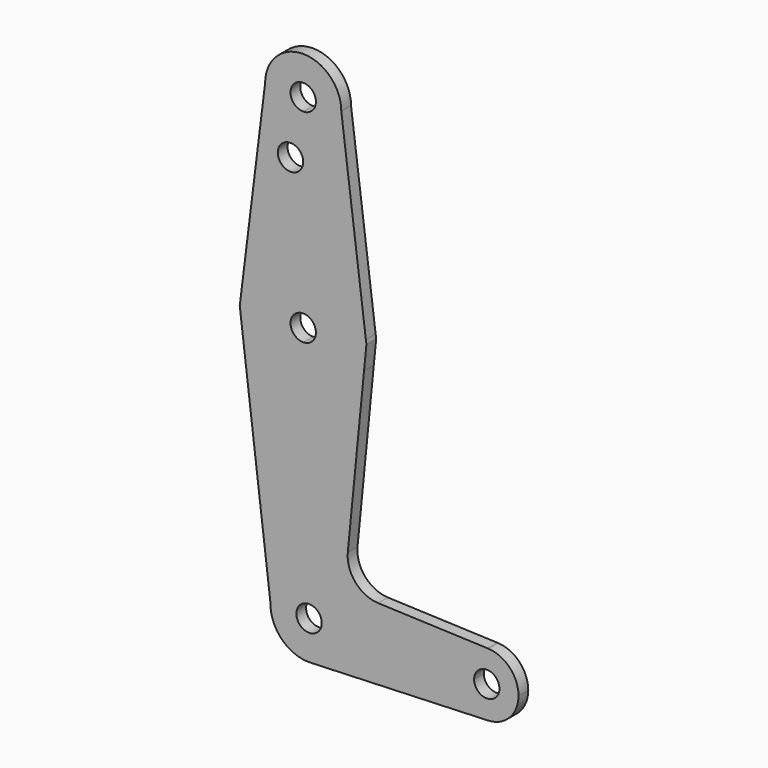
from build123d import *

# Parameters (mm, degrees)
F0_R     = 3.175
F1_DEPTH = 3.048


with BuildPart() as f1:
    # F0 (on Front) → F1 (new body)
    with BuildSketch(Plane.XZ):
        with BuildLine():
            ThreePointArc((-40.2117882118, -46.0434157276), (-37.9195183152, -46.9467537328), (-36.9635307828, -49.2175704733))
            Line((-36.9635307828, -49.2175704733), (-30.4929387527, -49.2175704733))
            ThreePointArc((-30.4929387527, -49.2175704733), (-33.3972114214, -42.3188706769), (-40.3610855146, -39.5745463105))
            Line((-40.3610855146, -39.5745463105), (-40.2117882118, -46.0434157276))
        make_face()
        with BuildLine():
            Line((-30.4929387527, -49.2175704733), (-36.9635307828, -49.2175704733))
            ThreePointArc((-36.9635307828, -49.2175704733), (-42.3575432504, -51.4883872137), (-40.2117882118, -46.0434157276))
            Line((-40.2117882118, -46.0434157276), (-40.3610855146, -39.5745463105))
            ThreePointArc((-40.3610855146, -39.5745463105), (-46.9764555291, -42.4146129712), (-49.7825692087, -49.0444564898))
            ThreePointArc((-49.7825692087, -49.0444564898), (-46.7848835913, -56.2078093787), (-39.4795413303, -58.8406250046))
            ThreePointArc((-39.4795413303, -58.8406250046), (-33.0889283464, -55.8009245652), (-30.4929387527, -49.2175704733))
        make_face()
        with BuildLine():
            ThreePointArc((-40.3610855146, -39.5745463105), (-33.3972114214, -42.3188706769), (-30.4929387527, -49.2175704733))
            Line((-30.4929387527, -49.2175704733), (-3.6260307828, -49.2175704733))
            ThreePointArc((-3.6260307828, -49.2175704733), (-1.2243575174, -43.5291147413), (4.5272992617, -41.2830053534))
            Line((4.5272992617, -41.2830053534), (-22.8459084544, -40.2300400931))
            ThreePointArc((-22.8459084544, -40.2300400931), (-28.5326050858, -37.5104766919), (-30.452220219, -31.5063429983))
            Line((-30.452220219, -31.5063429983), (-26.3874033783, 9.7581951748))
            ThreePointArc((-26.3874033783, 9.7581951748), (-31.9659630039, 1.6680517084), (-41.2377823768, -1.5883442013))
            Line((-41.2377823768, -1.5883442013), (-40.3610855146, -39.5745463105))
        make_face()
        with BuildLine():
            Line((-3.6260307828, -49.2175704733), (-30.4929387527, -49.2175704733))
            ThreePointArc((-30.4929387527, -49.2175704733), (-33.0889283464, -55.8009245652), (-39.4795413303, -58.8406250046))
            Line((-39.4795413303, -58.8406250046), (4.6157088211, -57.1492376696))
            ThreePointArc((4.6157088211, -57.1492376696), (-1.1925749502, -54.9367840602), (-3.6260307828, -49.2175704733))
        make_face()
        with BuildLine():
            ThreePointArc((-49.7825692087, -49.0444564898), (-46.9764555291, -42.4146129712), (-40.3610855146, -39.5745463105))
            Line((-40.3610855146, -39.5745463105), (-41.2377823768, -1.5883442013))
            ThreePointArc((-41.2377823768, -1.5883442013), (-51.3557623371, 1.7556537149), (-57.0797223857, 10.7440975125))
            Line((-57.0797223857, 10.7440975125), (-49.7825692087, -49.0444564898))
        make_face()
        with BuildLine():
            ThreePointArc((4.5272992617, -41.2830053534), (-1.2243575174, -43.5291147413), (-3.6260307828, -49.2175704733))
            ThreePointArc((-3.6260307828, -49.2175704733), (-1.1925749502, -54.9367840602), (4.6157088211, -57.1492376696))
            ThreePointArc((4.6157088211, -57.1492376696), (10.0306828042, -54.7216146407), (12.2489692172, -49.2175704733))
            ThreePointArc((12.2489692172, -49.2175704733), (10.0618609106, -43.7461079976), (4.705812903, -41.2898722381))
            Line((4.705812903, -41.2898722381), (4.5272992617, -41.2830053534))
        make_face()
        with BuildLine():
            ThreePointArc((7.480460495, -49.2175704733), (4.3114692172, -52.386561751), (1.1424779394, -49.2175704733))
            ThreePointArc((1.1424779394, -49.2175704733), (4.3114692172, -46.0485791955), (7.480460495, -49.2175704733))
        make_face(mode=Mode.SUBTRACT)
        with BuildLine():
            Line((-41.530812093, 11.1082747811), (-41.2377823768, -1.5883442013))
            ThreePointArc((-41.2377823768, -1.5883442013), (-31.9659630039, 1.6680517084), (-26.3874033783, 9.7581951748))
            Line((-26.3874033783, 9.7581951748), (-25.797109695, 15.7506413739))
            Line((-25.797109695, 15.7506413739), (-25.9336119369, 16.8225838675))
            ThreePointArc((-25.9336119369, 16.8225838675), (-31.3159532016, 26.372519997), (-41.6040695218, 30.1574295267))
            Line((-41.6040695218, 30.1574295267), (-41.604069522, 17.4574295267))
            ThreePointArc((-41.604069522, 17.4574295267), (-39.3590054917, 16.527493557), (-38.429069522, 14.2824295267))
            ThreePointArc((-38.429069522, 14.2824295267), (-39.3332527816, 12.0634170591), (-41.530812093, 11.1082747811))
        make_face()
        with BuildLine():
            ThreePointArc((-57.0797223857, 10.7440975125), (-51.3557623371, 1.7556537149), (-41.2377823768, -1.5883442013))
            Line((-41.2377823768, -1.5883442013), (-41.530812093, 11.1082747811))
            ThreePointArc((-41.530812093, 11.1082747811), (-44.7788582014, 14.2457983742), (-41.604069522, 17.4574295267))
            Line((-41.604069522, 17.4574295267), (-41.6040695218, 30.1574295267))
            ThreePointArc((-41.6040695218, 30.1574295267), (-51.2458107034, 26.8940294249), (-56.9234751411, 18.4455337145))
            Line((-56.9234751411, 18.4455337145), (-57.4764627709, 13.9947534011))
            Line((-57.4764627709, 13.9947534011), (-57.0797223857, 10.7440975125))
        make_face()
        with BuildLine():
            Line((-51.1290695215, 65.0824294972), (-56.9234751411, 18.4455337145))
            ThreePointArc((-56.9234751411, 18.4455337145), (-51.2458107034, 26.8940294249), (-41.6040695218, 30.1574295267))
            Line((-41.6040695218, 30.1574295267), (-41.6040695216, 50.8076295267))
            Line((-41.6040695216, 50.8076295267), (-41.6040695216, 55.5574295267))
            ThreePointArc((-41.6040695216, 55.5574295267), (-48.3392616018, 58.3472374255), (-51.1290695215, 65.0824294972))
        make_face()
        with Locations((-44.7790695216, 50.8076295267)):
            Circle(F0_R, mode=Mode.SUBTRACT)
        with BuildLine():
            ThreePointArc((-41.6040695218, 30.1574295267), (-31.3159532016, 26.372519997), (-25.9336119369, 16.8225838675))
            Line((-25.9336119369, 16.8225838675), (-32.0790695215, 65.0824295268))
            ThreePointArc((-32.0790695215, 65.0824295267), (-34.8688774307, 58.3472374359), (-41.6040695216, 55.5574295267))
            Line((-41.6040695216, 55.5574295267), (-41.6040695216, 50.8076295267))
            Line((-41.6040695216, 50.8076295267), (-41.6040695218, 30.1574295267))
        make_face()
        with BuildLine():
            ThreePointArc((-32.0790695215, 65.0824295267), (-41.6040695362, 74.6074295267), (-51.1290695215, 65.0824294972))
            ThreePointArc((-51.1290695215, 65.0824294972), (-48.3392616018, 58.3472374255), (-41.6040695216, 55.5574295267))
            ThreePointArc((-41.6040695216, 55.5574295267), (-34.8688774307, 58.3472374359), (-32.0790695215, 65.0824295267))
        make_face()
        with BuildLine():
            ThreePointArc((-38.4290695215, 65.0824295267), (-39.3590054912, 62.8373654965), (-41.6040695215, 61.9074295267))
            ThreePointArc((-41.6040695215, 61.9074295267), (-43.8491335517, 67.327493557), (-38.4290695215, 65.0824295267))
        make_face(mode=Mode.SUBTRACT)
    extrude(amount=F1_DEPTH)


solid = f1.part
